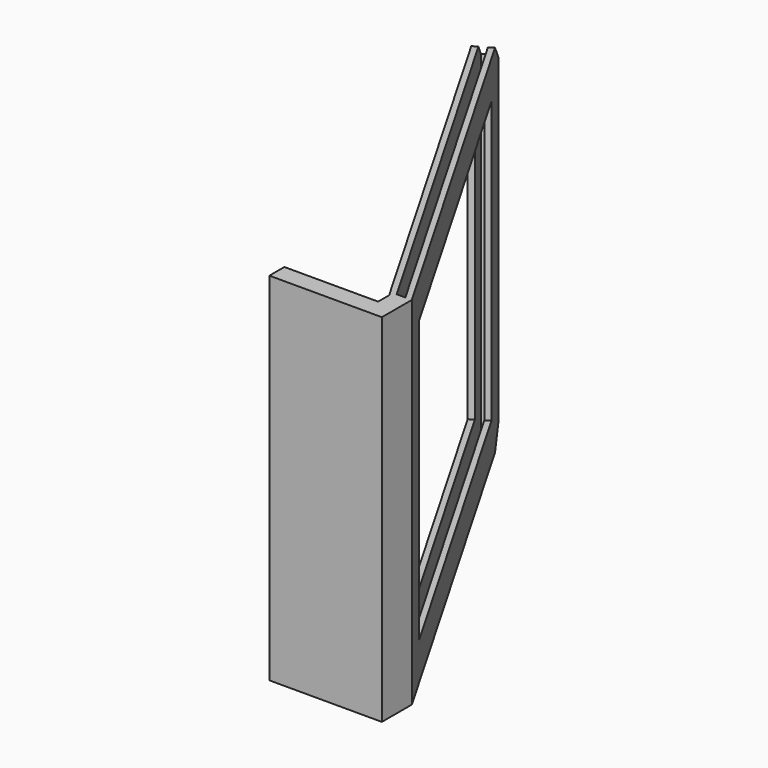
from build123d import *

# Parameters (mm, degrees)
F1_DEPTH    = 241.3
F2_W        = 254
F2_H        = 190.5
F3_DEPTH    = 25.4
F5_DEPTH    = 508
F6_T1_DEPTH = 78.0207478943
F7_T1_DEPTH = 78.0207478943


# Not quite as in the source:
# - a fillet or chamfer that OpenCascade refuses, or shapes differently, is made with other operations: its cross-section is extruded or revolved along the edge and cut away or added


with BuildPart() as f1:
    # F0 (on Top) → F1 (new body)
    with BuildSketch(Plane.XY):
        Polygon((0, 12.7), (0, 0), (76.2, 0), (76.2, 25.4), (-76.2, 289.3645430735), (-87.1985226281, 283.0145430735), (63.5, 21.9970452561), (63.5, 12.7), align=None)
    extrude(amount=F1_DEPTH)

    # F2 (on face) → F3 (cut)
    with BuildSketch(Plane(origin=(68.1485226281, 39.3455678842, 0), x_dir=(-0.5, 0.8660254038, 0), z_dir=(0.8660254038, 0.5, 0))):
        with Locations((136.2970452561, 120.65)):
            Rectangle(F2_W, F2_H)
    extrude(amount=-F3_DEPTH, mode=Mode.SUBTRACT)

    # F4 (on face) → F5 (cut)
    with BuildSketch(Plane.XY.offset(241.3)):
        Polygon((-81.9939685629, 281.6199870148), (65.9347099118, 25.4), (71.8005932508, 25.4), (-77.5945560587, 284.1599890084), align=None)
    extrude(amount=-F5_DEPTH, mode=Mode.SUBTRACT)

    # F6: chamfer of 12.7 on 1 edges, made by hand

    # F6_s2 → F6_t1 (cut)
    with BuildSketch(Plane(origin=(96.4332361634, 55.6757548578, 0), x_dir=(0, 0, 1), z_dir=(-0.8660254038, -0.5, 0))):
        Polygon((0, 275.9970452561), (12.7, 288.6970452561), (0, 288.6970452561), align=None)
    extrude(amount=F6_T1_DEPTH, mode=Mode.SUBTRACT)

    # F7: chamfer of 12.7 on 1 edges, made by hand

    # F7_s2 → F7_t1 (cut)
    with BuildSketch(Plane(origin=(96.4332361634, 55.6757548578, 0), x_dir=(0, 0, 1), z_dir=(-0.8660254038, -0.5, 0))):
        Polygon((241.3, 275.9970452561), (228.6, 288.6970452561), (241.3, 288.6970452561), align=None)
    extrude(amount=F7_T1_DEPTH, mode=Mode.SUBTRACT)


solid = f1.part
